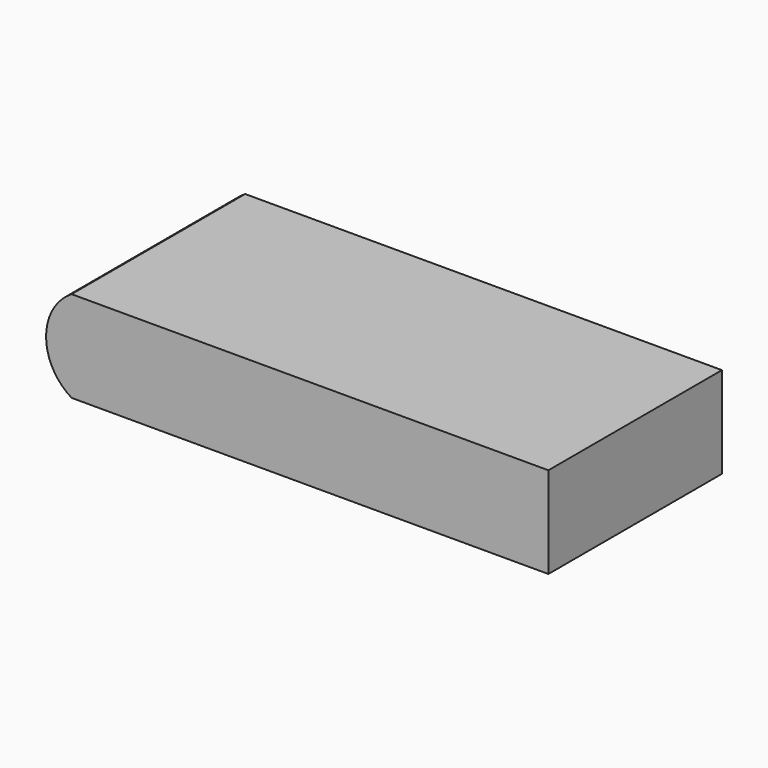
from build123d import *

# Parameters (mm, degrees)
F1_DEPTH       = 9.5
F2_TEXT_SIZE   = 1.3556315227
F2_TEXT_SIZE_2 = 1.452462877
F2_TEXT_SIZE_3 = 3.9700632139
F3_DEPTH       = 0.5


# Not quite as in the source:
# - Text() gives the source's letters only with a copy of the font that has no kerning and outlines rounded to 1/6400 em; it was checked with that copy


with BuildPart() as f1:
    # F0 (on Front) → F1 (new body, symmetric)
    with BuildSketch(Plane.XZ):
        with BuildLine():
            Line((22, -4), (22, 4))
            Line((22, 4), (-19.7646824203, 4))
            ThreePointArc((-19.7646824203, 4), (-21.4032601081, 2.2911047926), (-22, 0))
            ThreePointArc((-22, 0), (-21.4032601081, -2.2911047926), (-19.7646824203, -4))
            Line((-19.7646824203, -4), (22, -4))
        make_face()
    extrude(amount=F1_DEPTH, both=True)

    # F2 (on face) → F3 (join)
    with BuildSketch(Plane(origin=(0, 0, -4), x_dir=(1, 0, 0), z_dir=(0, 0, -1))):
        with Locations((3.9637088776, 6.3834171742)):
            Text('Li-poly RC Battery', F2_TEXT_SIZE, font='Open Sans', font_style=FontStyle.BOLD, text_align=(TextAlign.LEFT, TextAlign.BOTTOM))
        with Locations((0.8263937198, 4.3615889736)):
            Text('HIGH POWER HIGH QUALITY', F2_TEXT_SIZE_2, font='Open Sans', text_align=(TextAlign.LEFT, TextAlign.BOTTOM))
        with Locations((0.8263927302, -3.1679759268)):
            Text('7.4V 25C', F2_TEXT_SIZE_3, font='Open Sans', text_align=(TextAlign.LEFT, TextAlign.BOTTOM))
        with Locations((0.8263927302, -8.5672618976)):
            Text('1000mAh', F2_TEXT_SIZE_3, font='Open Sans', text_align=(TextAlign.LEFT, TextAlign.BOTTOM))
    extrude(amount=F3_DEPTH)


solid = f1.part
